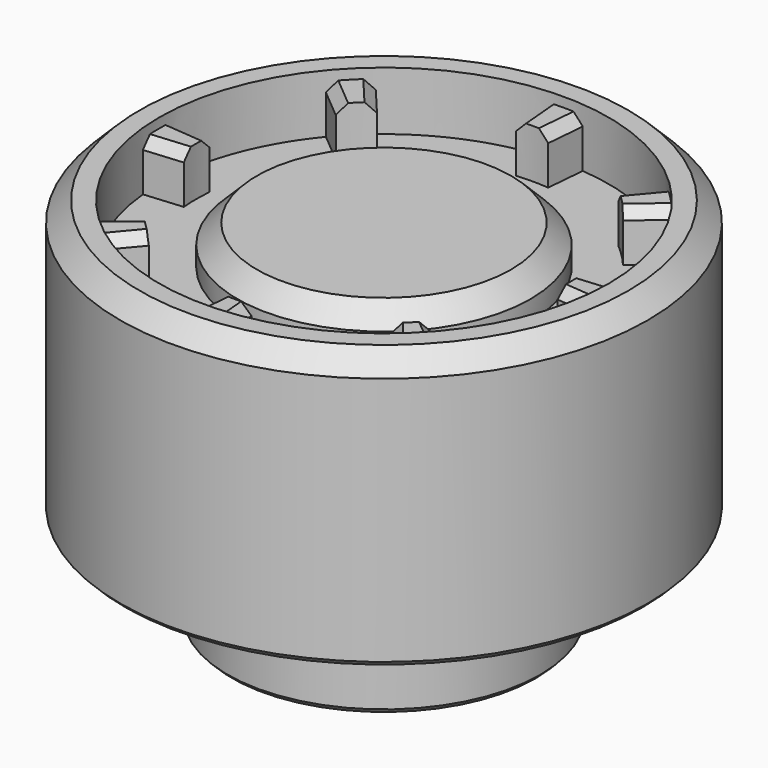
from build123d import *

# Parameters (mm, degrees)
F3_DEPTH = 2.5
F4_SIZE  = 1
F5_SIZE  = 0.5
F6_SIZE  = 0.25


# Not quite as in the source:
# - a feature names something its author has since deleted; it is built from what else it names


with BuildPart() as f1:
    # F0 (on Front) → F1 (revolve)
    with BuildSketch(Plane.XZ):
        Polygon((7, 15), (7, 0), (8, 0), (8, 5), (13.5, 5), (13.5, 19), (11.5, 19), (11.5, 16), (7.5, 16), (7.5, 18), (0, 18), (0, 15), align=None)
    revolve(axis=Axis((0, 0, 16.5), (0, 0, 1)))

    # F2 (on face) → F3 (join)
    with BuildSketch(Plane.XY.offset(16)):
        with BuildLine():
            Line((0.8279795561, 9.4638496319), (1.0022910416, 11.4562390281))
            ThreePointArc((1.0022910416, 11.4562390281), (0, 11.5), (-1.0022910416, 11.4562390281))
            Line((-1.0022910416, 11.4562390281), (-0.8279795561, 9.4638496319))
            ThreePointArc((-0.8279795561, 9.4638496319), (0, 9.5), (0.8279795561, 9.4638496319))
        make_face()
        with BuildLine():
            ThreePointArc((8.8304981344, 7.3669737816), (8.1575715841, 8.1058019869), (7.4230424297, 8.7834185308))
            Line((7.4230424297, 8.7834185308), (6.1641167123, 7.2830892843))
            ThreePointArc((6.1641167123, 7.2830892843), (6.7751488416, 6.723181496), (7.3350566299, 6.1121493667))
            Line((7.3350566299, 6.1121493667), (8.8304981344, 7.3669737816))
        make_face()
        with BuildLine():
            ThreePointArc((11.5, 0), (11.4899071638, 0.4816984201), (11.4596463708, 0.9625513265))
            Line((11.4596463708, 0.9625513265), (9.5662449685, 0.7969001683))
            ThreePointArc((9.5662449685, 0.7969001683), (9.6023953367, -0.0310793878), (9.5662449685, -0.8590589439))
            Line((9.5662449685, -0.8590589439), (11.4542973626, -1.0242421245))
            ThreePointArc((11.4542973626, -1.0242421245), (11.4885686591, -0.5126306323), (11.5, 0))
        make_face()
        with BuildLine():
            ThreePointArc((7.4117695743, -8.7929330588), (8.141359766, -8.1220847792), (8.810476783, -7.3909064976))
            Line((8.810476783, -7.3909064976), (7.385484621, -6.1951961001))
            ThreePointArc((7.385484621, -6.1951961001), (6.8255768326, -6.8062282293), (6.2145447034, -7.3661360177))
            Line((6.2145447034, -7.3661360177), (7.4117695743, -8.7929330588))
        make_face()
        with BuildLine():
            Line((-0.7566636072, -9.5973243563), (-0.9199020931, -11.4631487881))
            ThreePointArc((-0.9199020931, -11.4631487881), (0.0710446065, -11.4997805485), (1.0614630688, -11.450908093))
            Line((1.0614630688, -11.450908093), (0.899295505, -9.5973243563))
            ThreePointArc((0.899295505, -9.5973243563), (0.0713159489, -9.6334747244), (-0.7566636072, -9.5973243563))
        make_face()
        with BuildLine():
            Line((-7.263740681, -6.2456240912), (-8.7349008301, -7.4800740296))
            ThreePointArc((-8.7349008301, -7.4800740296), (-8.0552507812, -8.2074926044), (-7.3152358724, -8.8734054416))
            Line((-7.3152358724, -8.8734054416), (-6.0928007634, -7.4165640088))
            ThreePointArc((-6.0928007634, -7.4165640088), (-6.7038328927, -6.8566562204), (-7.263740681, -6.2456240912))
        make_face()
        with BuildLine():
            Line((-9.4949290196, 0.7255842194), (-11.464890553, 0.8979335212))
            ThreePointArc((-11.464890553, 0.8979335212), (-11.4995475928, -0.1020056943), (-11.4471576619, -1.1011727676))
            Line((-11.4471576619, -1.1011727676), (-9.4949290196, -0.9303748928))
            ThreePointArc((-9.4949290196, -0.9303748928), (-9.5310793878, -0.1023953367), (-9.4949290196, 0.7255842194))
        make_face()
        with BuildLine():
            ThreePointArc((-11.4471576619, -1.1011727676), (-11.4995475928, -0.1020056943), (-11.464890553, 0.8979335212))
            Line((-11.464890553, 0.8979335212), (-11.4873184158, 0.8998957049))
            ThreePointArc((-11.4873184158, 0.8998957049), (-11.5310793878, -0.1023953367), (-11.4873184158, -1.1046863783))
            Line((-11.4873184158, -1.1046863783), (-11.4471576619, -1.1011727676))
        make_face()
        with BuildLine():
            Line((-6.1432287545, 7.2326612933), (-7.4288039739, 8.7647501795))
            ThreePointArc((-7.4288039739, 8.7647501795), (-8.1684744461, 8.0869670673), (-8.8462575583, 7.347296595))
            Line((-8.8462575583, 7.347296595), (-7.3141686721, 6.0617213757))
            ThreePointArc((-7.3141686721, 6.0617213757), (-6.7542608837, 6.6727535049), (-6.1432287545, 7.2326612933))
        make_face()
    extrude(amount=F3_DEPTH)

    # F4
    f4_edges = [f1.edges().sort_by_distance(p)[0] for p in [
        (-13.5, 0, 19),
        (-7.5, 0, 18),
    ]]
    chamfer(f4_edges, length=F4_SIZE)

    # F5
    f5_edges = [f1.edges().sort_by_distance(p)[0] for p in [
        (-10.471043, -1.015774, 18.5),
        (-10.47991, 0.811759, 18.5),
        (-8.080213, 6.704509, 18.5),
        (-6.786016, 7.998706, 18.5),
        (-0.915135, 10.460044, 18.5),
        (0.915135, 10.460044, 18.5),
        (-6.704018, -8.144985, 18.5),
        (-7.999321, -6.862849, 18.5),
        (0.980379, -10.524116, 18.5),
        (-0.838283, -10.530237, 18.5),
        (8.097981, -6.793051, 18.5),
        (6.813157, -8.079535, 18.5),
        (10.512946, 0.879726, 18.5),
        (10.510271, -0.941651, 18.5),
        (8.082777, 6.739562, 18.5),
        (6.79358, 8.033254, 18.5),
    ]]
    chamfer(f5_edges, length=F5_SIZE)

    # F6
    f6_edges = [f1.edges().sort_by_distance(p)[0] for p in [
        (-13.5, 0, 5),
        (-8, 0, 5),
        (-8, 0, 0),
    ]]
    chamfer(f6_edges, length=F6_SIZE)


solid = f1.part
